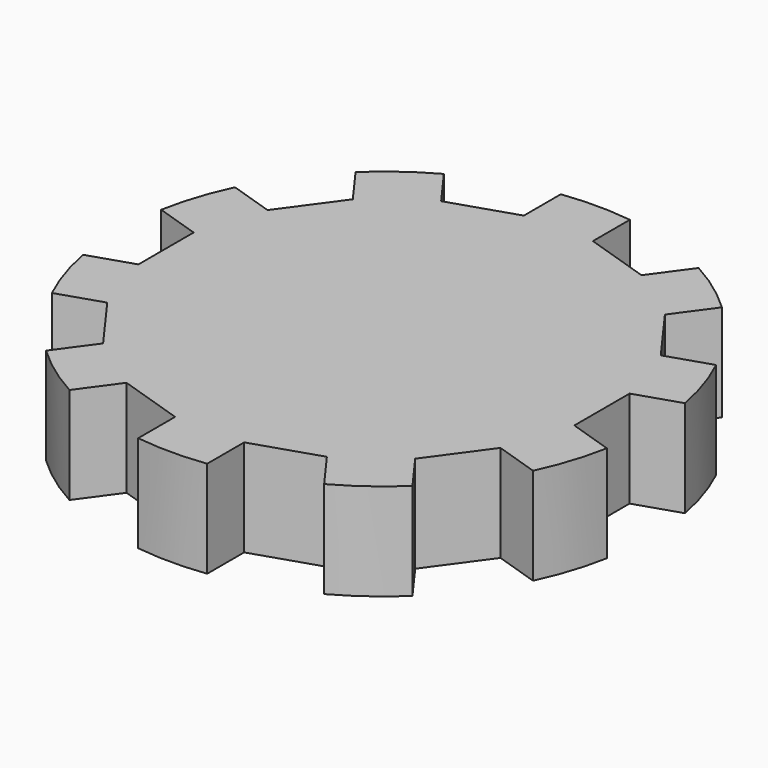
from build123d import *

# Parameters (mm, degrees)
F0_R     = 139.7
F1_DEPTH = 50.8
F3_DEPTH = 50.801


with BuildPart() as f1:
    # F0 (on Top) → F1 (new body)
    with BuildSketch(Plane.XY):
        Circle(F0_R)
    extrude(amount=F1_DEPTH)

    # F2 (on face) → F3 (intersect, through all)
    with BuildSketch(Plane.XY.offset(50.8)):
        with BuildLine():
            Line((-81.829765289, 81.829765289), (-52.537943385, 103.1115196251))
            Line((-52.537943385, 103.1115196251), (-66.7753086177, 122.7075717265))
            ThreePointArc((-66.7753086177, 122.7075717265), (-82.1135997453, 113.0196741142), (-96.0671305217, 101.4258173904))
            Line((-96.0671305217, 101.4258173905), (-81.829765289, 81.829765289))
        make_face()
        with BuildLine():
            Line((-18.1033415291, 114.3), (18.1033415291, 114.3))
            Line((18.1033415291, 114.3), (18.1033415291, 138.522052488))
            ThreePointArc((18.1033415291, 138.522052488), (0, 139.7), (-18.1033415291, 138.522052488))
            Line((-18.1033415291, 138.522052488), (-18.1033415291, 114.3))
        make_face()
        with BuildLine():
            Line((52.537943385, 103.1115196251), (81.829765289, 81.829765289))
            Line((81.829765289, 81.829765289), (96.0671305217, 101.4258173905))
            ThreePointArc((96.0671305217, 101.4258173904), (82.1135997453, 113.0196741142), (66.7753086177, 122.7075717265))
            Line((66.7753086177, 122.7075717265), (52.537943385, 103.1115196251))
        make_face()
        with BuildLine():
            Line((103.1115196251, 52.537943385), (114.3, 18.1033415291))
            Line((114.3, 18.1033415291), (137.3365408567, 25.5883673865))
            ThreePointArc((137.3365408567, 25.5883673865), (132.8625953264, 43.1696741142), (126.1480604818, 60.0229692424))
            Line((126.1480604818, 60.0229692424), (103.1115196251, 52.537943385))
        make_face()
        with BuildLine():
            Line((137.3365408567, -25.5883673865), (114.3, -18.1033415291))
            Line((114.3, -18.1033415291), (103.1115196251, -52.537943385))
            Line((103.1115196251, -52.537943385), (126.1480604818, -60.0229692424))
            ThreePointArc((126.1480604818, -60.0229692424), (132.8625953264, -43.1696741142), (137.3365408567, -25.5883673865))
        make_face()
        with BuildLine():
            Line((96.0671305217, -101.4258173905), (81.829765289, -81.829765289))
            Line((81.829765289, -81.829765289), (52.537943385, -103.1115196251))
            Line((52.537943385, -103.1115196251), (66.7753086177, -122.7075717265))
            ThreePointArc((66.7753086177, -122.7075717265), (82.1135997453, -113.0196741142), (96.0671305217, -101.4258173904))
        make_face()
        with BuildLine():
            Line((18.1033415291, -138.522052488), (18.1033415291, -114.3))
            Line((18.1033415291, -114.3), (-18.1033415291, -114.3))
            Line((-18.1033415291, -114.3), (-18.1033415291, -138.522052488))
            ThreePointArc((-18.1033415291, -138.522052488), (0, -139.7), (18.1033415291, -138.522052488))
        make_face()
        with BuildLine():
            Line((-66.7753086177, -122.7075717265), (-52.537943385, -103.1115196251))
            Line((-52.537943385, -103.1115196251), (-81.829765289, -81.829765289))
            Line((-81.829765289, -81.829765289), (-96.0671305217, -101.4258173905))
            ThreePointArc((-96.0671305217, -101.4258173904), (-82.1135997453, -113.0196741142), (-66.7753086177, -122.7075717265))
        make_face()
        with BuildLine():
            Line((-126.1480604818, -60.0229692424), (-103.1115196251, -52.537943385))
            Line((-103.1115196251, -52.537943385), (-114.3, -18.1033415291))
            Line((-114.3, -18.1033415291), (-137.3365408567, -25.5883673865))
            ThreePointArc((-137.3365408567, -25.5883673865), (-132.8625953264, -43.1696741142), (-126.1480604818, -60.0229692424))
        make_face()
        with BuildLine():
            Line((-114.3, 18.1033415291), (-103.1115196251, 52.537943385))
            Line((-103.1115196251, 52.537943385), (-126.1480604818, 60.0229692424))
            ThreePointArc((-126.1480604818, 60.0229692424), (-132.8625953264, 43.1696741142), (-137.3365408567, 25.5883673865))
            Line((-137.3365408567, 25.5883673865), (-114.3, 18.1033415291))
        make_face()
        Polygon((114.3, -18.1033415291), (114.3, 18.1033415291), (103.1115196251, 52.537943385), (81.829765289, 81.829765289), (52.537943385, 103.1115196251), (18.1033415291, 114.3), (-18.1033415291, 114.3), (-52.537943385, 103.1115196251), (-81.829765289, 81.829765289), (-103.1115196251, 52.537943385), (-114.3, 18.1033415291), (-114.3, -18.1033415291), (-103.1115196251, -52.537943385), (-81.829765289, -81.829765289), (-52.537943385, -103.1115196251), (-18.1033415291, -114.3), (18.1033415291, -114.3), (52.537943385, -103.1115196251), (81.829765289, -81.829765289), (103.1115196251, -52.537943385), align=None)
    extrude(amount=-F3_DEPTH, mode=Mode.INTERSECT)


solid = f1.part
